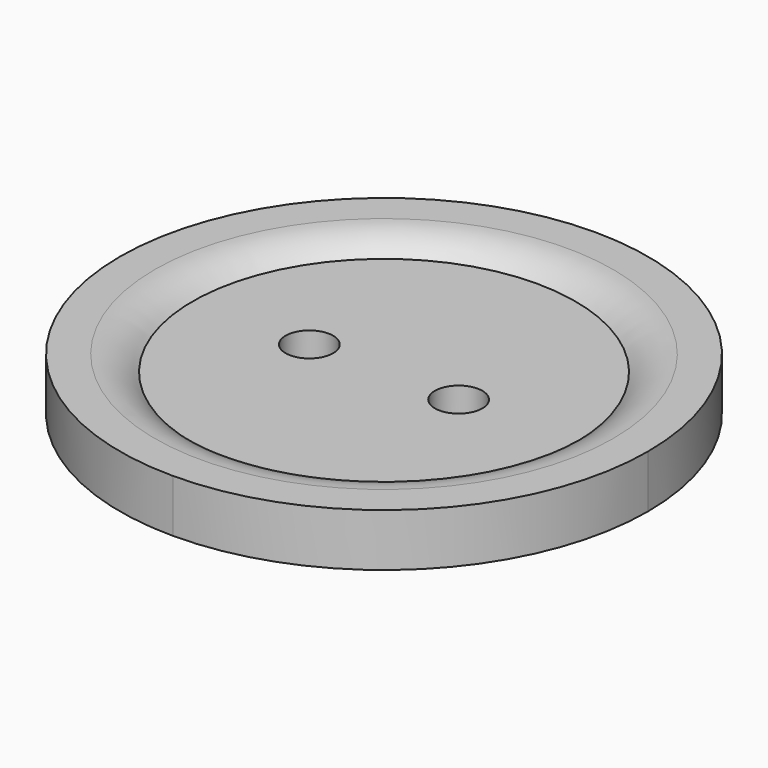
from build123d import *

# Parameters (mm, degrees)
F1_DEPTH = 5.08
F0_R     = 2.286
F2_DEPTH = 3.556


# Not quite as in the source:
# - a fillet or chamfer that OpenCascade refuses, or shapes differently, is made with other operations: its cross-section is extruded or revolved along the edge and cut away or added


with BuildPart() as f1:
    # F0 (on Top) → F1 (new body)
    with BuildSketch(Plane.XY):
        with BuildLine():
            ThreePointArc((0, -25.4), (17.9605122421, -17.9605122421), (25.4, 0))
            ThreePointArc((25.4, 0), (17.9605122421, 17.9605122421), (0, 25.4))
            Line((0, 25.4), (0, 18.415))
            ThreePointArc((0, 18.415), (13.0213713756, 13.0213713756), (18.415, 0))
            ThreePointArc((18.415, 0), (13.0213713756, -13.0213713756), (0, -18.415))
            Line((0, -18.415), (0, -25.4))
        make_face()
        with BuildLine():
            Line((0, 18.415), (0, 25.4))
            ThreePointArc((0, 25.4), (-25.4, 0), (0, -25.4))
            Line((0, -25.4), (0, -18.415))
            ThreePointArc((0, -18.415), (-18.415, 0), (0, 18.415))
        make_face()
    extrude(amount=F1_DEPTH)

    # F0 (on Top) → F2 (join)
    with BuildSketch(Plane.XY):
        with BuildLine():
            Line((0, -18.415), (0, 18.415))
            ThreePointArc((0, 18.415), (-18.415, 0), (0, -18.415))
        make_face()
        with Locations((-7.1823259524, 0)):
            Circle(F0_R, mode=Mode.SUBTRACT)
        with BuildLine():
            ThreePointArc((18.415, 0), (13.0213713756, 13.0213713756), (0, 18.415))
            Line((0, 18.415), (0, -18.415))
            ThreePointArc((0, -18.415), (13.0213713756, -13.0213713756), (18.415, 0))
        make_face()
        with Locations((7.1823259524, 0)):
            Circle(F0_R, mode=Mode.SUBTRACT)
    extrude(amount=F2_DEPTH)

    # F3: fillet of radius 5.08 on 1 edges, made by hand

    # F3_s1 → F3_t2 (revolve, cut)
    with BuildSketch(Plane.XZ):
        with BuildLine():
            ThreePointArc((22.0428456417, 5.08), (20.0753701018, 4.6835285843), (18.415, 3.556))
            Line((18.415, 3.556), (18.415, 5.08))
            Line((18.415, 5.08), (22.0428456417, 5.08))
        make_face()
    revolve(axis=Axis((0, 0, 5.08), (0, 0, -1)), mode=Mode.SUBTRACT)


solid = f1.part
